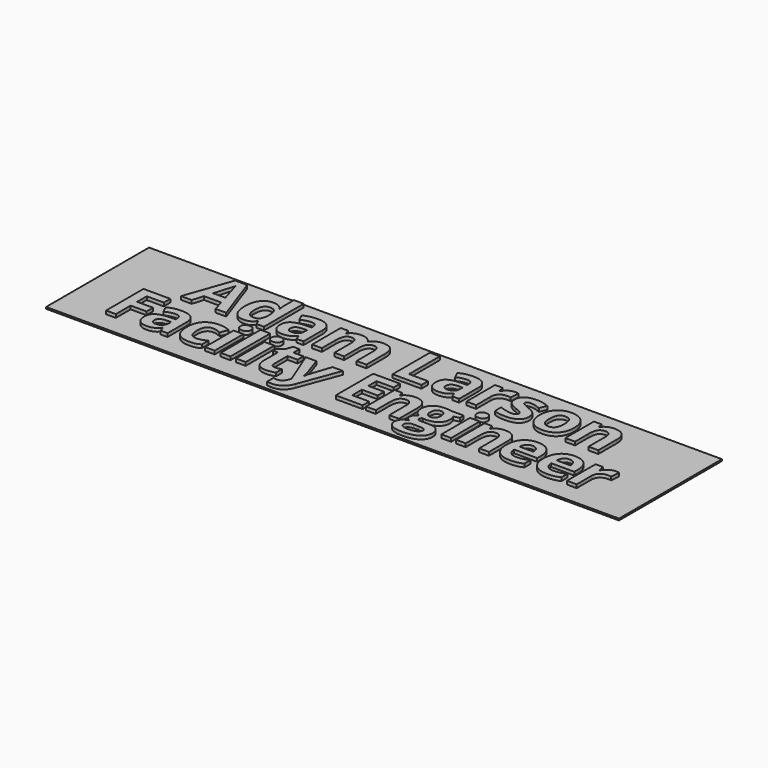
from build123d import *

# Parameters (mm, degrees)
F0_TEXT_SIZE = 24.6944444444
F1_DEPTH     = 1.27
F2_W         = 216
F2_H         = 48.514
F3_DEPTH     = 0.635


# Not quite as in the source:
# - Text() gives the source's letters only with a copy of the font that has no kerning and outlines rounded to 1/6400 em; it was checked with that copy


with BuildPart() as f1:
    # F0 (on Top) → F1 (new body)
    with BuildSketch(Plane.XY):
        with Locations((-33.5361261333, -11.5835723103)):
            Text('A', F0_TEXT_SIZE, font='Open Sans', font_style=FontStyle.BOLD, text_align=(TextAlign.LEFT, TextAlign.BOTTOM))
        with Locations((-15.9961803868, -11.5835723103)):
            Text('d', F0_TEXT_SIZE, font='Open Sans', font_style=FontStyle.BOLD, text_align=(TextAlign.LEFT, TextAlign.BOTTOM))
        with Locations((-0.4301365499, -11.5835723103)):
            Text('a', F0_TEXT_SIZE, font='Open Sans', font_style=FontStyle.BOLD, text_align=(TextAlign.LEFT, TextAlign.BOTTOM))
        with Locations((13.9472115403, -11.5835723103)):
            Text('m', F0_TEXT_SIZE, font='Open Sans', font_style=FontStyle.BOLD, text_align=(TextAlign.LEFT, TextAlign.BOTTOM))
        with Locations((43.9947831549, -11.5835723103)):
            Text('L', F0_TEXT_SIZE, font='Open Sans', font_style=FontStyle.BOLD, text_align=(TextAlign.LEFT, TextAlign.BOTTOM))
        with Locations((58.2438634501, -11.5835723103)):
            Text('a', F0_TEXT_SIZE, font='Open Sans', font_style=FontStyle.BOLD, text_align=(TextAlign.LEFT, TextAlign.BOTTOM))
        with Locations((72.1245665751, -11.5835723103)):
            Text('r', F0_TEXT_SIZE, font='Open Sans', font_style=FontStyle.BOLD, text_align=(TextAlign.LEFT, TextAlign.BOTTOM))
        with Locations((83.2343104987, -11.5835723103)):
            Text('s', F0_TEXT_SIZE, font='Open Sans', font_style=FontStyle.BOLD, text_align=(TextAlign.LEFT, TextAlign.BOTTOM))
        with Locations((95.1474506896, -11.5835723103)):
            Text('o', F0_TEXT_SIZE, font='Open Sans', font_style=FontStyle.BOLD, text_align=(TextAlign.LEFT, TextAlign.BOTTOM))
        with Locations((-47.2521261333, -32.5385723103)):
            Text('F', F0_TEXT_SIZE, font='Open Sans', font_style=FontStyle.BOLD, text_align=(TextAlign.LEFT, TextAlign.BOTTOM))
        with Locations((-34.918684293, -32.5385723103)):
            Text('a', F0_TEXT_SIZE, font='Open Sans', font_style=FontStyle.BOLD, text_align=(TextAlign.LEFT, TextAlign.BOTTOM))
        with Locations((-21.0184130256, -32.5385723103)):
            Text('c', F0_TEXT_SIZE, font='Open Sans', font_style=FontStyle.BOLD, text_align=(TextAlign.LEFT, TextAlign.BOTTOM))
        with Locations((-9.6881829909, -32.5385723103)):
            Text('i', F0_TEXT_SIZE, font='Open Sans', font_style=FontStyle.BOLD, text_align=(TextAlign.LEFT, TextAlign.BOTTOM))
        with Locations((-3.7612958381, -32.5385723103)):
            Text('l', F0_TEXT_SIZE, font='Open Sans', font_style=FontStyle.BOLD, text_align=(TextAlign.LEFT, TextAlign.BOTTOM))
        with Locations((1.9958170091, -32.5385723103)):
            Text('i', F0_TEXT_SIZE, font='Open Sans', font_style=FontStyle.BOLD, text_align=(TextAlign.LEFT, TextAlign.BOTTOM))
        with Locations((8.8118695264, -32.5385723103)):
            Text('t', F0_TEXT_SIZE, font='Open Sans', font_style=FontStyle.BOLD, text_align=(TextAlign.LEFT, TextAlign.BOTTOM))
        with Locations((19.4494975646, -32.5385723103)):
            Text('y', F0_TEXT_SIZE, font='Open Sans', font_style=FontStyle.BOLD, text_align=(TextAlign.LEFT, TextAlign.BOTTOM))
        with Locations((109.401988016, -11.5835723103)):
            Text('n', F0_TEXT_SIZE, font='Open Sans', font_style=FontStyle.BOLD, text_align=(TextAlign.LEFT, TextAlign.BOTTOM))
        with Locations((39.3387228251, -32.5385723103)):
            Text('E', F0_TEXT_SIZE, font='Open Sans', font_style=FontStyle.BOLD, text_align=(TextAlign.LEFT, TextAlign.BOTTOM))
        with Locations((51.037440273, -32.5385723103)):
            Text('n', F0_TEXT_SIZE, font='Open Sans', font_style=FontStyle.BOLD, text_align=(TextAlign.LEFT, TextAlign.BOTTOM))
        with Locations((65.3624229119, -32.5385723103)):
            Text('g', F0_TEXT_SIZE, font='Open Sans', font_style=FontStyle.BOLD, text_align=(TextAlign.LEFT, TextAlign.BOTTOM))
        with Locations((79.4658170091, -32.5385723103)):
            Text('i', F0_TEXT_SIZE, font='Open Sans', font_style=FontStyle.BOLD, text_align=(TextAlign.LEFT, TextAlign.BOTTOM))
        with Locations((84.946440273, -32.5385723103)):
            Text('n', F0_TEXT_SIZE, font='Open Sans', font_style=FontStyle.BOLD, text_align=(TextAlign.LEFT, TextAlign.BOTTOM))
        with Locations((99.3389467834, -32.5385723103)):
            Text('e', F0_TEXT_SIZE, font='Open Sans', font_style=FontStyle.BOLD, text_align=(TextAlign.LEFT, TextAlign.BOTTOM))
        with Locations((113.3089467834, -32.5385723103)):
            Text('e', F0_TEXT_SIZE, font='Open Sans', font_style=FontStyle.BOLD, text_align=(TextAlign.LEFT, TextAlign.BOTTOM))
        with Locations((126.790018832, -32.5385723103)):
            Text('r', F0_TEXT_SIZE, font='Open Sans', font_style=FontStyle.BOLD, text_align=(TextAlign.LEFT, TextAlign.BOTTOM))
    extrude(amount=F1_DEPTH)

    # F2 (on Top) → F3 (join)
    with BuildSketch(Plane.XY):
        with Locations((46.2279153598, -15.6415530395)):
            Rectangle(F2_W, F2_H)
    extrude(amount=-F3_DEPTH)


solid = f1.part
